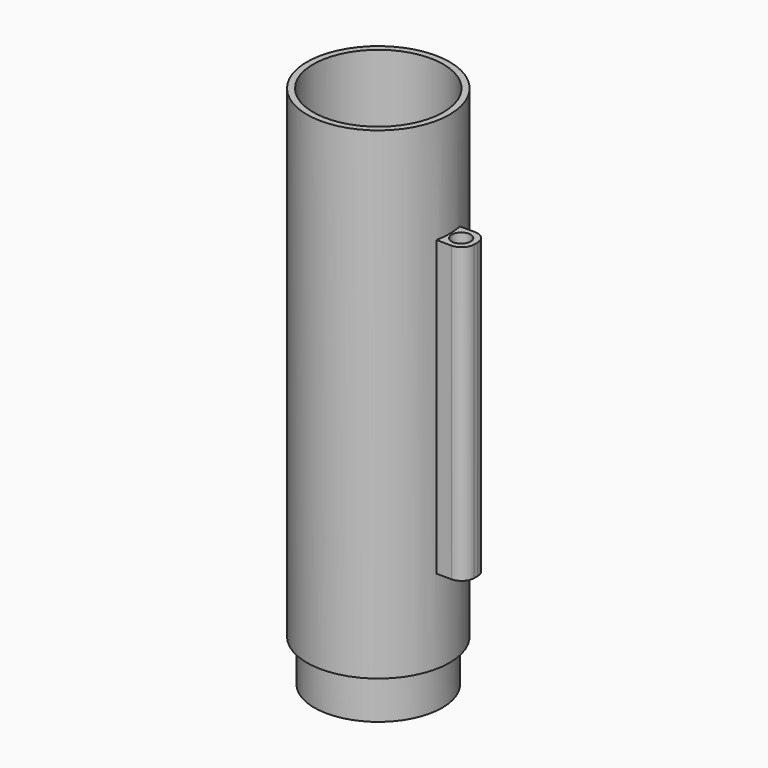
from build123d import *

# Parameters (mm, degrees)
F1_R     = 17
F1_R_2   = 15.5
F2_DEPTH = 115
F3_R     = 17
F4_DEPTH = 2
F5_R     = 15.25
F6_DEPTH = 10
F8_R     = 2.25
F9_DEPTH = 70


# Not quite as in the source:
# - a feature of the source that left no trace in its solid (it failed there, or was rolled back) is left out


with BuildPart() as f2:
    # F1 (on offset) → F2 (new body)
    with BuildSketch(Plane.XY.offset(107)):
        Circle(F1_R)
        Circle(F1_R_2, mode=Mode.SUBTRACT)
    extrude(amount=F2_DEPTH)

    # F3 (on offset) → F4 (join)
    with BuildSketch(Plane.XY.offset(107)):
        Circle(F3_R)
    extrude(amount=F4_DEPTH)

    # F5 (on face) → F6 (join)
    with BuildSketch(Plane(origin=(0, 0, 107), x_dir=(1, 0, 0), z_dir=(0, 0, -1))):
        Circle(F5_R)
    extrude(amount=F6_DEPTH)

    # F8 (on offset) → F9 (join)
    with BuildSketch(Plane.XY.offset(127)):
        with BuildLine():
            Line((20.2600458013, 3.5), (16.2600458013, 3.5))
            Line((16.2600458013, 3.5), (16.2600458013, -3.5))
            Line((16.2600458013, -3.5), (20.2600458013, -3.5))
            ThreePointArc((20.2600458013, -3.5), (22.3813661449, -2.6213203436), (23.2600458013, -0.5))
            Line((23.2600458013, -0.5), (23.2600458013, 0.5))
            ThreePointArc((23.2600458013, 0.5), (22.3813661449, 2.6213203436), (20.2600458013, 3.5))
        make_face()
        with Locations((19.7600458013, 0)):
            Circle(F8_R, mode=Mode.SUBTRACT)
    extrude(amount=F9_DEPTH)


solid = f2.part
